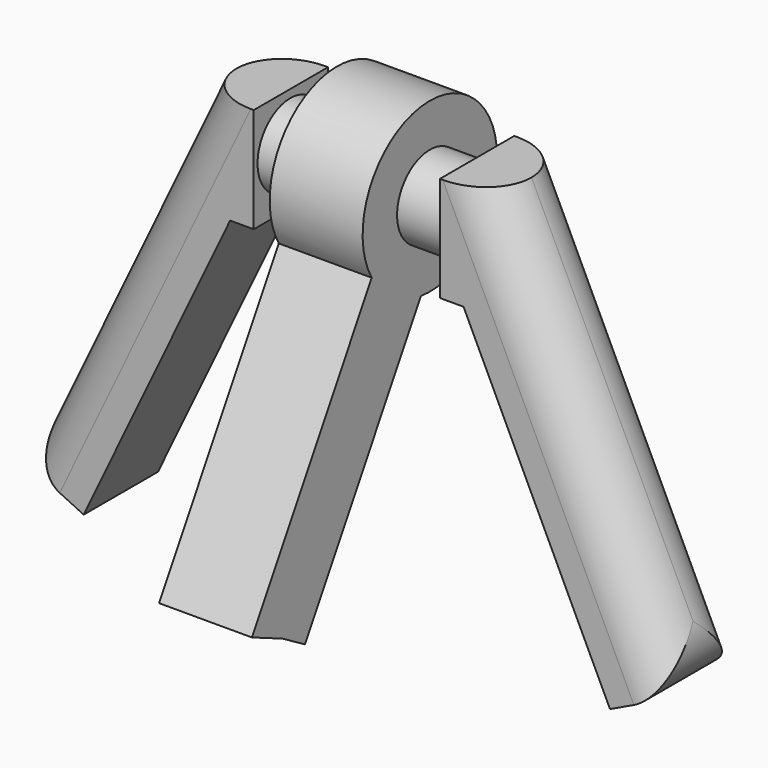
from build123d import *

# Parameters (mm, degrees)
F1_DEPTH = 10
F3_DEPTH = 10.01716
F4_R     = 4.99999
F6_DEPTH = 5


# Not quite as in the source:
# - a fillet or chamfer is up to 0.001 mm smaller than in the source, because OpenCascade refuses the exact size


with BuildPart() as f1:
    # F0 (on Front) → F1 (new body)
    with BuildSketch(Plane.XZ):
        Polygon((-12.5626804332, 29.607558623), (0, 29.607558623), (0, 40.9011654556), (-15.8720966429, 40.9011654556), (-35.4069806635, 0), (-28.3201927203, -3.3847343715), align=None)
    extrude(amount=F1_DEPTH)

    # F2 (on face) → F3 (cut)
    with BuildSketch(Plane.YZ):
        Polygon((-10, 29.607558623), (-8.6038469049, 29.607558623), (0, 29.607558623), (0, 40.9011654556), (-10, 40.9011654556), align=None)
        with BuildLine():
            ThreePointArc((-7.3082493459, 31.8197726236), (-7.2727253308, 39.4503255628), (-0.6703296735, 35.6247574091))
            ThreePointArc((-0.6703296735, 35.6247574091), (-2.8869450444, 31.7991892554), (-7.3082493459, 31.8197726236))
        make_face(mode=Mode.SUBTRACT)
    extrude(amount=-F3_DEPTH, mode=Mode.SUBTRACT)

    # F4 (radius 5 in the source; OpenCascade refuses exactly that, so slightly less here)
    f4_edges = [f1.edges().sort_by_distance(p)[0] for p in [
        (-25.639539, -10, 20.450583),
        (-25.639539, 0, 20.450583),
        (-35.406981, -5, 0),
    ]]
    fillet(f4_edges, radius=F4_R)

    # F5: F1 across face


with BuildPart() as f1_1:
    add(f1.part)
    add(f1.part.mirror(Plane(origin=(0, -5.0798351876, 35.6247574091), x_dir=(0, 1, 0), z_dir=(1, 0, 0))))


with BuildPart() as f6:
    # F2 (on face) → F6 (new body, symmetric)
    with BuildSketch(Plane.YZ):
        with BuildLine():
            ThreePointArc((-12.9000592681, 31.0769466924), (-11.4864525822, 29.2377596368), (-9.6516098344, 27.8185186501))
            ThreePointArc((-9.6516098344, 27.8185186501), (-8.0214187442, 27.0699007087), (-6.2755623418, 26.6576662667))
            ThreePointArc((-6.2755623418, 26.6576662667), (0.8792497216, 28.8183050271), (3.9666274903, 35.6247574091))
            ThreePointArc((3.9666274903, 35.6247574091), (-7.4349489542, 44.3592823607), (-12.9000592681, 31.0769466924))
        make_face()
        Polygon((0, 29.607558623), (-8.6038469049, 29.607558623), (-10, 29.607558623), (-10, 40.9011654556), (0, 40.9011654556), align=None, mode=Mode.SUBTRACT)
        with BuildLine():
            Line((-24.9078488827, 1.768712223), (-9.6516098344, 27.8185186501))
            ThreePointArc((-9.6516098344, 27.8185186501), (-11.4864525822, 29.2377596368), (-12.9000592681, 31.0769466924))
            Line((-12.9000592681, 31.0769466924), (-29.0196302747, 3.553013495))
            Line((-29.0196302747, 3.553013495), (-24.9078488827, 1.768712223))
        make_face()
        with BuildLine():
            ThreePointArc((-6.2755623418, 26.6576662667), (-8.0214187442, 27.0699007087), (-9.6516098344, 27.8185186501))
            Line((-9.6516098344, 27.8185186501), (-24.9078488827, 1.768712223))
            Line((-24.9078488827, 1.768712223), (-21.8877984701, 0))
            Line((-21.8877984701, 0), (-6.2755623418, 26.6576662667))
        make_face()
        Polygon((-10, 29.607558623), (-8.6038469049, 29.607558623), (0, 29.607558623), (0, 40.9011654556), (-10, 40.9011654556), align=None)
        with BuildLine():
            ThreePointArc((-7.3082493459, 31.8197726236), (-7.2727253308, 39.4503255628), (-0.6703296735, 35.6247574091))
            ThreePointArc((-0.6703296735, 35.6247574091), (-2.8869450444, 31.7991892554), (-7.3082493459, 31.8197726236))
        make_face(mode=Mode.SUBTRACT)
    extrude(amount=F6_DEPTH, both=True)


solid = Compound([f1_1.part, f6.part])
